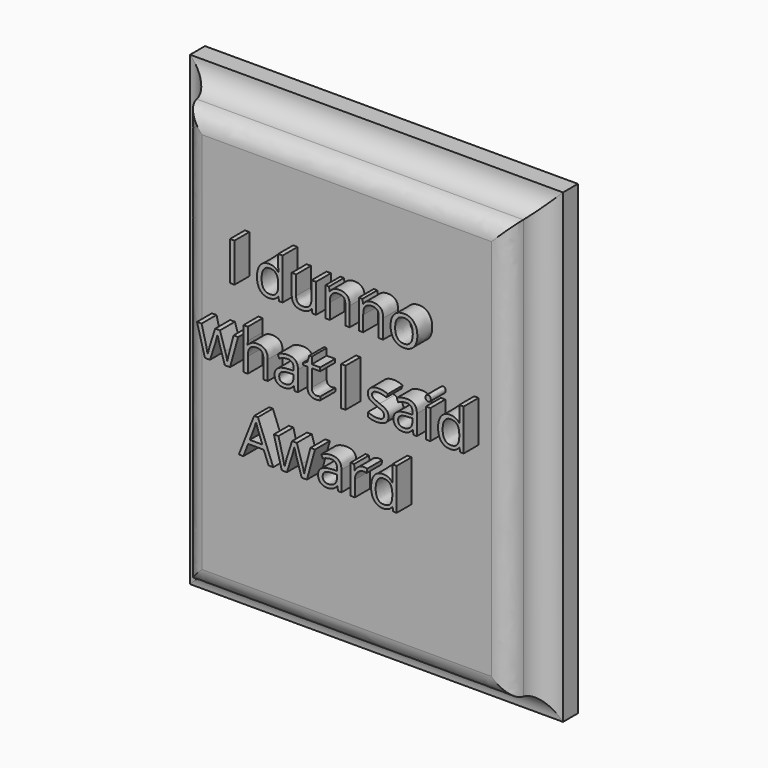
from build123d import *

# Parameters (mm, degrees)
F0_W         = 101.6
F0_H         = 127
F1_DEPTH     = 15.24
F2_W         = 101.6
F2_H         = 127
F2_W_2       = 88.9
F2_H_2       = 114.3
F3_DEPTH     = 10.16
F4_R         = 6.34999
F5_R         = 5.08
F6_TEXT_SIZE = 14.8288935022
F7_DEPTH     = 5.08


# Not quite as in the source:
# - a fillet or chamfer is up to 0.001 mm smaller than in the source, because OpenCascade refuses the exact size
# - Text() gives the source's letters only with a copy of the font that has no kerning and outlines rounded to 1/6400 em; it was checked with that copy


with BuildPart() as f1:
    # F0 (on Front) → F1 (new body)
    with BuildSketch(Plane.XZ):
        with Locations((-50.8, 63.5)):
            Rectangle(F0_W, F0_H)
    extrude(amount=F1_DEPTH)

    # F2 (on face) → F3 (cut)
    with BuildSketch(Plane.XZ.offset(15.24)):
        with Locations((-50.8, 63.5)):
            Rectangle(F2_W, F2_H)
        with Locations((-50.8, 63.5)):
            Rectangle(F2_W_2, F2_H_2, mode=Mode.SUBTRACT)
    extrude(amount=-F3_DEPTH, mode=Mode.SUBTRACT)

    # F4 (radius 6.35 in the source; OpenCascade refuses exactly that, so slightly less here)
    f4_edges = [f1.edges().sort_by_distance(p)[0] for p in [
        (-50.8, -5.08, 120.65),
        (-6.35, -5.08, 63.5),
        (-95.25, -5.08, 63.5),
        (-50.8, -5.08, 6.35),
    ]]
    fillet(f4_edges, radius=F4_R)

    # F5
    f5_edges = [f1.edges().sort_by_distance(p)[0] for p in [
        (-6.35, -15.24, 63.5),
        (-50.8, -15.24, 6.35),
        (-95.25, -15.24, 63.5),
        (-50.8, -15.24, 120.65),
    ]]
    fillet(f5_edges, radius=F5_R)

    # F6 (on face) → F7 (join)
    with BuildSketch(Plane.XZ.offset(15.24)):
        with Locations((-79.9943840824, 85.9139713527)):
            Text('I dunno', F6_TEXT_SIZE, font='Open Sans', text_align=(TextAlign.LEFT, TextAlign.BOTTOM))
        with Locations((-87.7007746743, 65.7466761898)):
            Text('what I said', F6_TEXT_SIZE, font='Open Sans', text_align=(TextAlign.LEFT, TextAlign.BOTTOM))
        with Locations((-76.1411887864, 45.5793810268)):
            Text('Award', F6_TEXT_SIZE, font='Open Sans', text_align=(TextAlign.LEFT, TextAlign.BOTTOM))
    extrude(amount=F7_DEPTH)


solid = f1.part
